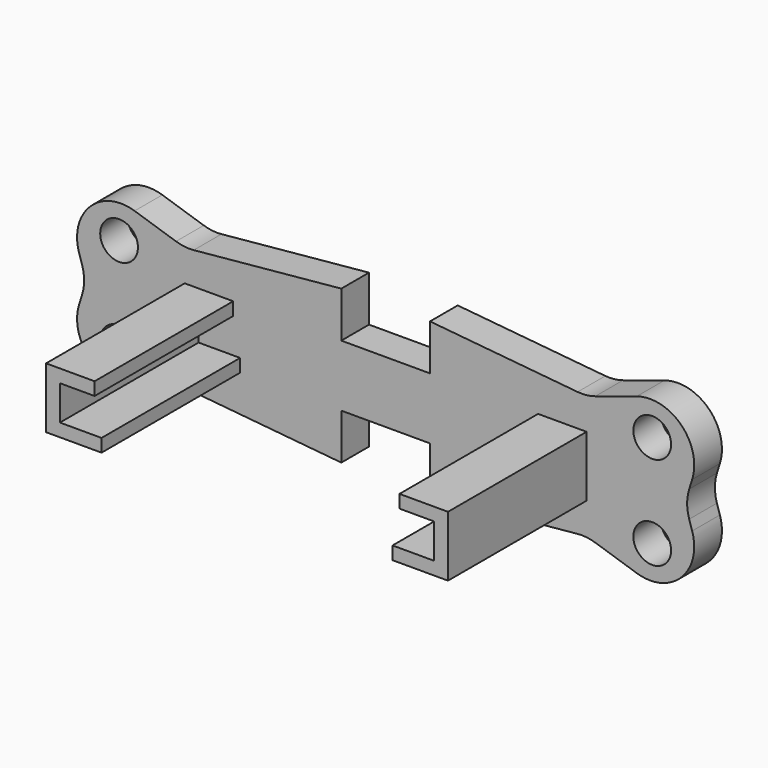
from build123d import *

# Parameters (mm, degrees)
F2_DEPTH = 30
F3_DEPTH = 5
F4_R     = 2.7226233937
F5_DEPTH = 5
F6_R     = 6.35


# Not quite as in the source:
# - a feature names something its author has since deleted; it is built from what else it names


with BuildPart() as f2:
    # F0 (on Front) → F2 (new body)
    with BuildSketch(Plane.XZ):
        Polygon((20.9966870546, -4.375), (28.9966870546, -4.375), (28.9966870546, 0), (28.0000005364, 0), (26.9966870546, 0), (26.9966870546, -2.5), (20.9966870546, -2.5), align=None)
        Polygon((28.0000005364, 0), (28.9966870546, 0), (28.9966870546, 4.375), (21.9966870546, 4.375), (21.9966870546, 2.5), (26.9966870546, 2.5), (26.9966870546, 0), align=None)
    extrude(amount=F2_DEPTH)


with BuildPart() as f2b:
    # F0 (on Front) → F2, piece 2 (new body)
    with BuildSketch(Plane.XZ):
        Polygon((-26.9966870546, -2.5), (-26.9966870546, 0), (-28.0000005364, 0), (-28.9966870546, 0), (-28.9966870546, -4.375), (-20.9966870546, -4.375), (-20.9966870546, -2.5), align=None)
        Polygon((-28.0000005364, 0), (-26.9966870546, 0), (-26.9966870546, 2.5), (-21.9966870546, 2.5), (-21.9966870546, 4.375), (-28.9966870546, 4.375), (-28.9966870546, 0), align=None)
    extrude(amount=F2_DEPTH)


with BuildPart() as f3:
    # F1 (on Front) → F3 (new body)
    with BuildSketch(Plane.XZ):
        Polygon((29, -8.8925119489), (29, 8.8925119489), (6.3987928443, 11.0501443781), (6.3987928443, 4.4462559745), (0, 4.4462559745), (-6.3987928443, 4.4462559745), (-6.3987928443, 11.0501443781), (-29, 8.8925119489), (-29, -8.8925119489), (-6.3987928443, -11.0501443781), (-6.3987928443, -4.4462559745), (0, -4.4462559745), (6.3987928443, -4.4462559745), (6.3987928443, -11.0501443781), align=None)
    extrude(amount=F3_DEPTH)

    # F4 (on face) → F5 (join)
    with BuildSketch(Plane(origin=(0, 0, 0), x_dir=(-1, 0, 0), z_dir=(0, 1, 0))):
        Polygon((-29, -8.8925119489), (-29, 8.8925119489), (-38.4654798061, 11.9462138973), (-47.9309596121, 14.9999158457), (-43.1982197091, 0), (-47.9309596121, -14.9999158457), (-38.4654798061, -11.9462138973), align=None)
        with Locations((-38.4654798061, -6.7365324358)):
            Circle(F4_R, mode=Mode.SUBTRACT)
        with Locations((-38.4654798061, 6.7365324358)):
            Circle(F4_R, mode=Mode.SUBTRACT)
        Polygon((38.4654798061, 11.9462138973), (29, 8.8925119489), (29, -8.8925119489), (47.9309596121, -14.9999158457), (43.1982197091, 0), (47.9309596121, 14.9999158457), align=None)
        with Locations((38.4654798061, -6.7365324358)):
            Circle(F4_R, mode=Mode.SUBTRACT)
        with Locations((38.4654798061, 6.7365324358)):
            Circle(F4_R, mode=Mode.SUBTRACT)
    extrude(amount=-F5_DEPTH)

    # F6
    f6_edges = [f3.edges().sort_by_distance(p)[0] for p in [
        (43.19822, -2.5, 0),
        (47.93096, -2.5, 14.999916),
        (47.93096, -2.5, -14.999916),
        (29, -2.5, -8.892512),
        (-29, -2.5, -8.892512),
        (-47.93096, -2.5, -14.999916),
        (-43.19822, -2.5, 0),
        (-47.93096, -2.5, 14.999916),
        (-29, -2.5, 8.892512),
        (29, -2.5, 8.892512),
    ]]
    fillet(f6_edges, radius=F6_R)


solid = Compound([f2.part, f2b.part, f3.part])
